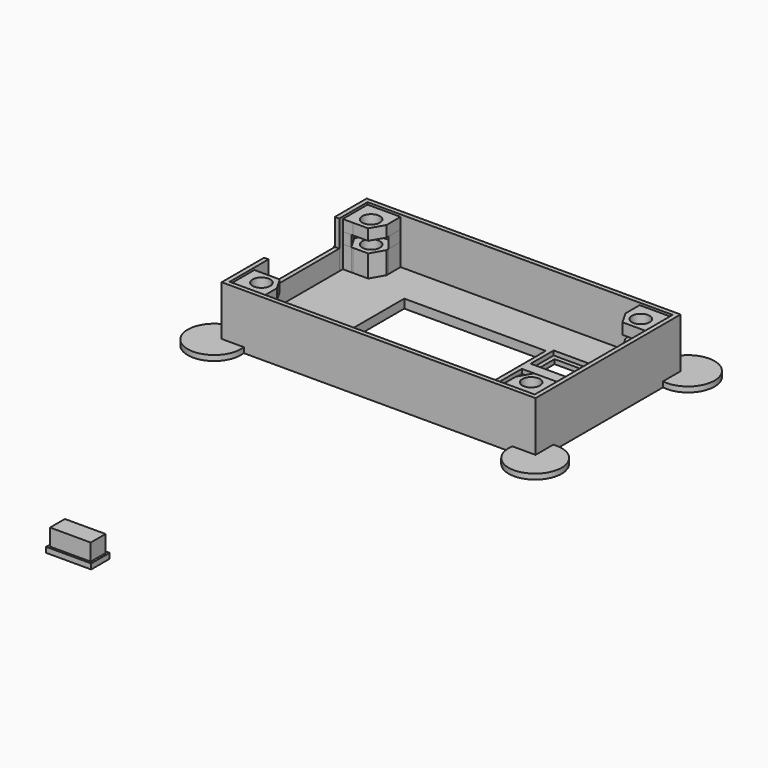
from build123d import *

# Parameters (mm, degrees)
F0_R      = 2
F1_DEPTH  = 7
F2_DEPTH  = 7
F3_DEPTH  = 2.5
F4_START  = 2.5
F1_FACE_R = 2
F4_DEPTH  = 2.5
F0_W      = 32
F0_H      = 23
F0_W_2    = 11.5
F0_H_2    = 6.5
F5_DEPTH  = 2
F0_W_3    = 9.5
F0_H_3    = 4.5
F6_DEPTH  = 1
F7_DEPTH  = 12.5
F0_W_4    = 1
F0_H_4    = 20
F8_DEPTH  = 6.5
F0_W_5    = 10.2
F0_H_5    = 5.2
F0_W_6    = 9.2
F0_H_6    = 4.2
F9_DEPTH  = 1.2
F10_DEPTH = 5
F11_DEPTH = 1.2


with BuildPart() as f1:
    # F0 (on Top) → F1 (new body)
    with BuildSketch(Plane.XY):
        Polygon((56.2425711751, 29.4110085815), (56.2425711751, 36.414245103), (54.3157895307, 36.414245103), (56.0530762776, 33.4181404888), (54.1540001392, 30.1145803152), (50.3434950368, 30.1074484079), (48.7784756274, 32.8064627658), (48.7784756274, 29.4110085815), (52.2425711751, 29.4110085815), align=None)
        Polygon((56.0530762776, 33.4181404888), (54.3157895307, 36.414245103), (53.9690040281, 36.414245103), (50.5049084804, 36.4077615509), (48.7784756274, 33.4045250294), (48.7784756274, 32.8064627658), (50.3434950368, 30.1074484079), (54.1540001392, 30.1145803152), align=None)
        with Locations((52.2425711751, 33.4110085815)):
            Circle(F0_R, mode=Mode.SUBTRACT)
    extrude(amount=F1_DEPTH)


with BuildPart() as f1b:
    # F0 (on Top) → F1, piece 2 (new body)
    with BuildSketch(Plane.XY):
        Polygon((-10.8411283625, 36.4077615509), (-12.7574288249, 36.4077615509), (-12.7574288249, 29.4110085815), (-5.2933332772, 29.4110085815), (-5.2933332772, 32.8155396842), (-6.8459998608, 30.1145803152), (-10.6565049632, 30.1074484079), (-12.5679339274, 33.4038766742), align=None)
        Polygon((-10.4950915196, 36.4077615509), (-10.8411283625, 36.4077615509), (-12.5679339274, 33.4038766742), (-10.6565049632, 30.1074484079), (-6.8459998608, 30.1145803152), (-5.2933332772, 32.8155396842), (-5.2933332772, 33.4174921336), (-7.0309959719, 36.414245103), align=None)
        with Locations((-8.7574288249, 33.4110085815)):
            Circle(F0_R, mode=Mode.SUBTRACT)
    extrude(amount=F1_DEPTH)


with BuildPart() as f1c:
    # F0 (on Top) → F1, piece 3 (new body)
    with BuildSketch(Plane.XY):
        Polygon((-5.2933332772, 68.4110085815), (-12.7574288249, 68.4110085815), (-12.7574288249, 61.40777206), (-10.8306471805, 61.40777206), (-12.5679339274, 64.4038766742), (-10.668857789, 67.7074368479), (-6.8583526866, 67.7145687551), (-5.2933332772, 65.0155543972), align=None)
        Polygon((-5.2933332772, 64.4174921336), (-5.2933332772, 65.0155543972), (-6.8583526866, 67.7145687551), (-10.668857789, 67.7074368479), (-12.5679339274, 64.4038766742), (-10.8306471805, 61.40777206), (-10.4838616779, 61.40777206), (-7.0197661302, 61.4142556121), align=None)
        with Locations((-8.7574288249, 64.4110085815)):
            Circle(F0_R, mode=Mode.SUBTRACT)
    extrude(amount=F1_DEPTH)


with BuildPart() as f1d:
    # F0 (on Top) → F1, piece 4 (new body)
    with BuildSketch(Plane.XY):
        Polygon((56.2425711751, 68.4110085815), (48.7784756274, 68.4110085815), (48.7784756274, 65.0064774788), (50.331142211, 67.7074368479), (54.1416473134, 67.7145687551), (56.0530762776, 64.4181404888), (54.3266434245, 61.4149039673), (56.2425711751, 61.4184899011), align=None)
        Polygon((50.331142211, 67.7074368479), (48.7784756274, 65.0064774788), (48.7784756274, 64.4045250294), (50.5161383221, 61.40777206), (53.9802338698, 61.4142556121), (54.3266434245, 61.4149039673), (56.0530762776, 64.4181404888), (54.1416473134, 67.7145687551), align=None)
        with Locations((52.2425711751, 64.4110085815)):
            Circle(F0_R, mode=Mode.SUBTRACT)
    extrude(amount=F1_DEPTH)


with BuildPart() as f2:
    # F0 (on Top) → F2 (new body, through all)
    with BuildSketch(Plane.XY):
        Polygon((56.2425711751, 29.4110085815), (56.2425711751, 36.414245103), (54.3157895307, 36.414245103), (56.0530762776, 33.4181404888), (54.1540001392, 30.1145803152), (50.3434950368, 30.1074484079), (48.7784756274, 32.8064627658), (48.7784756274, 29.4110085815), (52.2425711751, 29.4110085815), align=None)
    extrude(amount=F2_DEPTH)


with BuildPart() as f2b:
    # F0 (on Top) → F2, piece 2 (new body, through all)
    with BuildSketch(Plane.XY):
        Polygon((56.2425711751, 68.4110085815), (48.7784756274, 68.4110085815), (48.7784756274, 65.0064774788), (50.331142211, 67.7074368479), (54.1416473134, 67.7145687551), (56.0530762776, 64.4181404888), (54.3266434245, 61.4149039673), (56.2425711751, 61.4184899011), align=None)
    extrude(amount=F2_DEPTH)


with BuildPart() as f2c:
    # F0 (on Top) → F2, piece 3 (new body, through all)
    with BuildSketch(Plane.XY):
        Polygon((-5.2933332772, 68.4110085815), (-12.7574288249, 68.4110085815), (-12.7574288249, 61.40777206), (-10.8306471805, 61.40777206), (-12.5679339274, 64.4038766742), (-10.668857789, 67.7074368479), (-6.8583526866, 67.7145687551), (-5.2933332772, 65.0155543972), align=None)
    extrude(amount=F2_DEPTH)


with BuildPart() as f2d:
    # F0 (on Top) → F2, piece 4 (new body, through all)
    with BuildSketch(Plane.XY):
        Polygon((-10.8411283625, 36.4077615509), (-12.7574288249, 36.4077615509), (-12.7574288249, 29.4110085815), (-5.2933332772, 29.4110085815), (-5.2933332772, 32.8155396842), (-6.8459998608, 30.1145803152), (-10.6565049632, 30.1074484079), (-12.5679339274, 33.4038766742), align=None)
    extrude(amount=F2_DEPTH)


with BuildPart() as f3:
    # F3 (new): a face of the model
    f3_faces = [f2.part.faces().sort_by_distance(p)[0] for p in [
        (56.1402197979, 32.9126268423, 7),
    ]]
    extrude(f3_faces, amount=F3_DEPTH)

    # F1_face (on face) → F4 (join)
    with BuildSketch(Plane(origin=(52.8230493213, 32.5673462874, 7), x_dir=(1, 0, 0), z_dir=(0, 0, 1)).offset(F4_START)):
        Polygon((3.4195218538, -3.1563377059), (3.4195218538, 3.8468988156), (1.1459547068, 3.8468988156), (-2.3181408409, 3.8404152635), (-4.0445736939, 0.837178742), (-4.0445736939, -3.1563377059), align=None)
        with Locations((-0.5804781462, 0.8436622941)):
            Circle(F1_FACE_R, mode=Mode.SUBTRACT)
    extrude(amount=F4_DEPTH)


with BuildPart() as f3b:
    # F3#2 (new): a face of the model
    f3_2_faces = [f2d.part.faces().sort_by_distance(p)[0] for p in [
        (-11.7007240321, 31.7043432897, 7),
    ]]
    extrude(f3_2_faces, amount=F3_DEPTH)


with BuildPart() as f3c:
    # F3#3 (new): a face of the model
    f3_3_faces = [f2c.part.faces().sort_by_distance(p)[0] for p in [
        (-5.9873000269, 66.4164030753, 7),
    ]]
    extrude(f3_3_faces, amount=F3_DEPTH)


with BuildPart() as f3d:
    # F3#4 (new): a face of the model
    f3_4_faces = [f2b.part.faces().sort_by_distance(p)[0] for p in [
        (52.5105234013, 68.3087059901, 7),
    ]]
    extrude(f3_4_faces, amount=F3_DEPTH)


with BuildPart() as f4:
    # F1_face (on face) → F4, piece 2 (new body)
    with BuildSketch(Plane(origin=(52.8230493213, 32.5673462874, 7), x_dir=(1, 0, 0), z_dir=(0, 0, 1)).offset(F4_START)):
        Polygon((-65.5804781462, 3.8404152635), (-65.5804781462, -3.1563377059), (-58.1163825985, -3.1563377059), (-58.1163825985, 0.8501458462), (-59.8540452932, 3.8468988156), (-63.3181408409, 3.8404152635), align=None)
        with Locations((-61.5804781462, 0.8436622941)):
            Circle(F1_FACE_R, mode=Mode.SUBTRACT)
    extrude(amount=F4_DEPTH)


with BuildPart() as f4b:
    # F1_face (on face) → F4, piece 3 (new body)
    with BuildSketch(Plane(origin=(52.8230493213, 32.5673462874, 7), x_dir=(1, 0, 0), z_dir=(0, 0, 1)).offset(F4_START)):
        Polygon((-58.1163825985, 35.8436622941), (-65.5804781462, 35.8436622941), (-65.5804781462, 28.8404257726), (-63.3069109992, 28.8404257726), (-59.8428154515, 28.8469093247), (-58.1163825985, 31.8501458462), align=None)
        with Locations((-61.5804781462, 31.8436622941)):
            Circle(F1_FACE_R, mode=Mode.SUBTRACT)
    extrude(amount=F4_DEPTH)


with BuildPart() as f4c:
    # F1_face (on face) → F4, piece 4 (new body)
    with BuildSketch(Plane(origin=(52.8230493213, 32.5673462874, 7), x_dir=(1, 0, 0), z_dir=(0, 0, 1)).offset(F4_START)):
        Polygon((3.4195218538, 35.8436622941), (-4.0445736939, 35.8436622941), (-4.0445736939, 31.837178742), (-2.3069109992, 28.8404257726), (3.4195218538, 28.8511436137), align=None)
        with Locations((-0.5804781462, 31.8436622941)):
            Circle(F1_FACE_R, mode=Mode.SUBTRACT)
    extrude(amount=F4_DEPTH)


with BuildPart() as f5:
    # F0 (on Top) → F5 (new body)
    with BuildSketch(Plane.XY):
        Polygon((48.7784756274, 68.4110085815), (-5.2933332772, 68.4110085815), (-5.2933332772, 65.0155543972), (-5.2933332772, 64.4174921336), (-7.0197661302, 61.4142556121), (-10.4838616779, 61.40777206), (-10.8306471805, 61.40777206), (-12.7574288249, 61.40777206), (-12.7574288249, 60.4110085815), (-12.7574288249, 40.4110085815), (-12.7574288249, 36.4077615509), (-10.8411283625, 36.4077615509), (-10.4950915196, 36.4077615509), (-7.0309959719, 36.414245103), (-5.2933332772, 33.4174921336), (-5.2933332772, 32.8155396842), (-5.2933332772, 29.4110085815), (48.7784756274, 29.4110085815), (48.7784756274, 32.8064627658), (48.7784756274, 33.4045250294), (50.5049084804, 36.4077615509), (53.9690040281, 36.414245103), (54.3157895307, 36.414245103), (56.2425711751, 36.414245103), (56.2425711751, 61.4184899011), (54.3266434245, 61.4149039673), (53.9802338698, 61.4142556121), (50.5161383221, 61.40777206), (48.7784756274, 64.4045250294), (48.7784756274, 65.0064774788), align=None)
        with Locations((18.7425711751, 47.9110085815)):
            Rectangle(F0_W, F0_H, mode=Mode.SUBTRACT)
        with Locations((41.4925711751, 38.6610085815)):
            Rectangle(F0_W_2, F0_H_2, mode=Mode.SUBTRACT)
        with Locations((41.4925711751, 48.1610085815)):
            Rectangle(F0_W_2, F0_H_2, mode=Mode.SUBTRACT)
        with Locations((41.4925711751, 57.1610085815)):
            Rectangle(F0_W_2, F0_H_2, mode=Mode.SUBTRACT)
    extrude(amount=F5_DEPTH)

    # F0 (on Top) → F6 (join)
    with BuildSketch(Plane.XY):
        with Locations((41.4925711751, 57.1610085815)):
            Rectangle(F0_W_2, F0_H_2)
        with Locations((41.4925711751, 57.1610085815)):
            Rectangle(F0_W_3, F0_H_3, mode=Mode.SUBTRACT)
        with Locations((41.4925711751, 48.1610085815)):
            Rectangle(F0_W_2, F0_H_2)
        with Locations((41.4925711751, 48.1610085815)):
            Rectangle(F0_W_3, F0_H_3, mode=Mode.SUBTRACT)
        with Locations((41.4925711751, 38.6610085815)):
            Rectangle(F0_W_2, F0_H_2)
        with Locations((41.4925711751, 38.6610085815)):
            Rectangle(F0_W_3, F0_H_3, mode=Mode.SUBTRACT)
    extrude(amount=F6_DEPTH)


with BuildPart() as f5b:
    # F0 (on Top) → F5, piece 2 (new body)
    with BuildSketch(Plane.XY):
        with Locations((-8.7574288249, 64.4110085815)):
            Circle(F0_R)
    extrude(amount=F5_DEPTH)


with BuildPart() as f5c:
    # F0 (on Top) → F5, piece 3 (new body)
    with BuildSketch(Plane.XY):
        with Locations((52.2425711751, 64.4110085815)):
            Circle(F0_R)
    extrude(amount=F5_DEPTH)


with BuildPart() as f5d:
    # F0 (on Top) → F5, piece 4 (new body)
    with BuildSketch(Plane.XY):
        with Locations((52.2425711751, 33.4110085815)):
            Circle(F0_R)
    extrude(amount=F5_DEPTH)


with BuildPart() as f5e:
    # F0 (on Top) → F5, piece 5 (new body)
    with BuildSketch(Plane.XY):
        with Locations((-8.7574288249, 33.4110085815)):
            Circle(F0_R)
    extrude(amount=F5_DEPTH)


with BuildPart() as f7:
    # F0 (on Top) → F7 (new body)
    with BuildSketch(Plane.XY):
        with BuildLine():
            Line((-12.7574288249, 61.40777206), (-12.7574288249, 68.4110085815))
            Line((-12.7574288249, 68.4110085815), (-5.2933332772, 68.4110085815))
            Line((-5.2933332772, 68.4110085815), (48.7784756274, 68.4110085815))
            Line((48.7784756274, 68.4110085815), (56.2425711751, 68.4110085815))
            Line((56.2425711751, 68.4110085815), (56.2425711751, 61.4184899011))
            Line((56.2425711751, 61.4184899011), (56.2425711751, 36.414245103))
            Line((56.2425711751, 36.414245103), (56.2425711751, 29.4110085815))
            Line((56.2425711751, 29.4110085815), (52.2425711751, 29.4110085815))
            ThreePointArc((52.2425711751, 29.4110085815), (52.0955733964, 28.9164089663), (51.9916138982, 28.4110085815))
            Line((51.9916138982, 28.4110085815), (57.2425711751, 28.4110085815))
            Line((57.2425711751, 28.4110085815), (57.2425711751, 33.4181404888))
            Line((57.2425711751, 33.4181404888), (57.2425711751, 64.4181404888))
            Line((57.2425711751, 64.4181404888), (57.2425711751, 69.4110085815))
            Line((57.2425711751, 69.4110085815), (52.2425711751, 69.4110085815))
            Line((52.2425711751, 69.4110085815), (-8.7574288249, 69.4110085815))
            Line((-8.7574288249, 69.4110085815), (-13.7574288249, 69.4110085815))
            Line((-13.7574288249, 69.4110085815), (-13.7574288249, 64.4045250294))
            Line((-13.7574288249, 64.4045250294), (-13.7574288249, 60.4110085815))
            Line((-13.7574288249, 60.4110085815), (-12.7574288249, 60.4110085815))
            Line((-12.7574288249, 60.4110085815), (-12.7574288249, 61.40777206))
        make_face()
        with BuildLine():
            Line((-12.7574288249, 36.4077615509), (-12.7574288249, 40.4110085815))
            Line((-12.7574288249, 40.4110085815), (-13.7574288249, 40.4110085815))
            Line((-13.7574288249, 40.4110085815), (-13.7574288249, 33.4038766742))
            Line((-13.7574288249, 33.4038766742), (-13.7574288249, 28.4110085815))
            Line((-13.7574288249, 28.4110085815), (-8.7574288249, 28.4110085815))
            Line((-8.7574288249, 28.4110085815), (51.9916138982, 28.4110085815))
            ThreePointArc((51.9916138982, 28.4110085815), (52.0955733964, 28.9164089663), (52.2425711751, 29.4110085815))
            Line((52.2425711751, 29.4110085815), (48.7784756274, 29.4110085815))
            Line((48.7784756274, 29.4110085815), (-5.2933332772, 29.4110085815))
            Line((-5.2933332772, 29.4110085815), (-12.7574288249, 29.4110085815))
            Line((-12.7574288249, 29.4110085815), (-12.7574288249, 36.4077615509))
        make_face()
    extrude(amount=F7_DEPTH)

    # F0 (on Top) → F11 (join)
    with BuildSketch(Plane.XY):
        with BuildLine():
            Line((-13.7574288249, 28.4110085815), (-13.7574288249, 33.4038766742))
            ThreePointArc((-13.7574288249, 33.4038766742), (-18.9237187174, 23.2302020618), (-8.7574288249, 28.4110085815))
            Line((-8.7574288249, 28.4110085815), (-13.7574288249, 28.4110085815))
        make_face()
        with BuildLine():
            ThreePointArc((-8.7574288249, 69.4110085815), (-18.9316812756, 74.5720808603), (-13.7574288249, 64.4045250294))
            Line((-13.7574288249, 64.4045250294), (-13.7574288249, 69.4110085815))
            Line((-13.7574288249, 69.4110085815), (-8.7574288249, 69.4110085815))
        make_face()
        with BuildLine():
            ThreePointArc((57.2425711751, 64.4181404888), (62.4088610676, 74.5918151013), (52.2425711751, 69.4110085815))
            Line((52.2425711751, 69.4110085815), (57.2425711751, 69.4110085815))
            Line((57.2425711751, 69.4110085815), (57.2425711751, 64.4181404888))
        make_face()
        with BuildLine():
            Line((57.2425711751, 28.4110085815), (51.9916138982, 28.4110085815))
            ThreePointArc((51.9916138982, 28.4110085815), (62.0557427442, 23.1136946779), (57.2425711751, 33.4181404888))
            Line((57.2425711751, 33.4181404888), (57.2425711751, 28.4110085815))
        make_face()
    extrude(amount=F11_DEPTH)


with BuildPart() as f8:
    # F0 (on Top) → F8 (new body)
    with BuildSketch(Plane.XY):
        with Locations((-13.2574288249, 50.4110085815)):
            Rectangle(F0_W_4, F0_H_4)
    extrude(amount=F8_DEPTH)


with BuildPart() as f9:
    # F0 (on Top) → F9 (new body)
    with BuildSketch(Plane.XY):
        with Locations((16.7951593995, -50.4477024078)):
            Rectangle(F0_W_5, F0_H_5)
        with Locations((16.7951593995, -50.4477024078)):
            Rectangle(F0_W_6, F0_H_6, mode=Mode.SUBTRACT)
    extrude(amount=F9_DEPTH)

    # F0 (on Top) → F10 (join)
    with BuildSketch(Plane.XY):
        with Locations((16.7951593995, -50.4477024078)):
            Rectangle(F0_W_6, F0_H_6)
    extrude(amount=F10_DEPTH)


solid = Compound([f1.part, f1b.part, f1c.part, f1d.part, f2.part, f2b.part, f2c.part, f2d.part, f3.part, f3b.part, f3c.part, f3d.part, f4.part, f4b.part, f4c.part, f5.part, f5b.part, f5c.part, f5d.part, f5e.part, f7.part, f8.part, f9.part])
